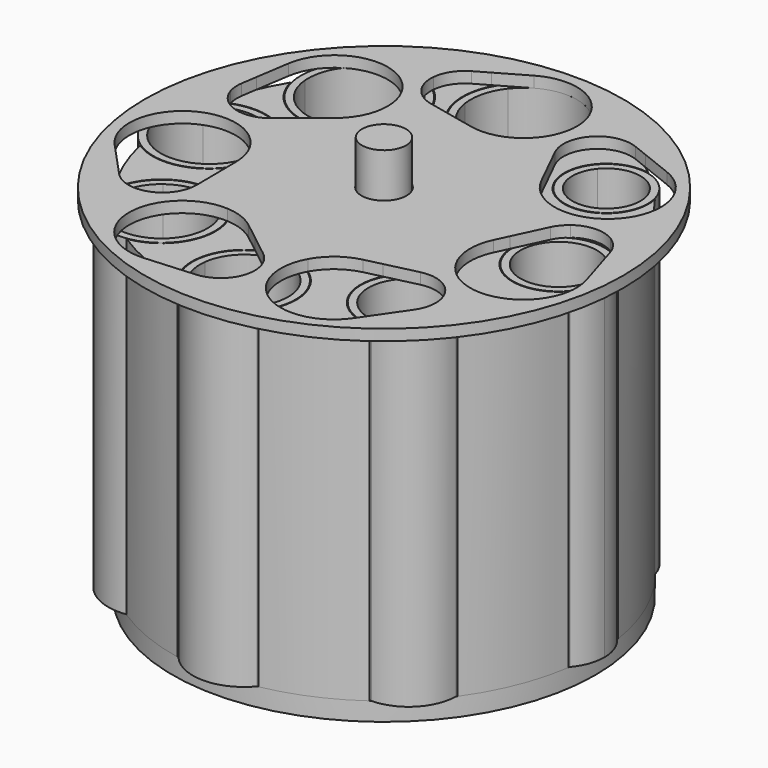
from build123d import *

# Parameters (mm, degrees)
F1_DEPTH = 90
F3_START = -90
F2_R     = 57.5
F2_R_2   = 6
F3_DEPTH = 5
F4_DEPTH = 90
F5_DEPTH = 88
F6_R     = 65
F6_R_2   = 6.125
F7_DEPTH = 3
F8_DEPTH = 15


with BuildPart() as f1:
    # F0 (on Top) → F1 (new body)
    with BuildSketch(Plane.XY):
        with BuildLine():
            ThreePointArc((45.8288421053, -12.4886841297), (34.9, 0), (45.8288421053, 12.4886841297))
            ThreePointArc((45.8288421053, 12.4886841297), (43.6591869219, 18.7116380181), (40.6490973012, 24.5743949793))
            ThreePointArc((40.6490973012, 24.5743949793), (25.4911994618, 25.4911994618), (24.5743949793, 40.6490973012))
            ThreePointArc((24.5743949793, 40.6490973012), (20.5775093162, 42.8114016396), (16.3922850173, 44.5818684211))
            ThreePointArc((16.3922850173, 44.5818684211), (0, 30.85), (-16.3922850173, 44.5818684211))
            ThreePointArc((-16.3922850173, 44.5818684211), (-18.4350753796, 43.7766832429), (-20.4384723604, 42.8779529312))
            ThreePointArc((-20.4384723604, 42.8779529312), (-22.2031529293, 22.2031529293), (-42.8779529312, 20.4384723604))
            ThreePointArc((-42.8779529312, 20.4384723604), (-44.0188706587, 17.8490623265), (-45.0035789474, 15.196311458))
            ThreePointArc((-45.0035789474, 15.196311458), (-32.1, 0), (-45.0035789474, -15.196311458))
            ThreePointArc((-45.0035789474, -15.196311458), (-43.7474044611, -18.5044481928), (-42.2484404987, -21.7098888857))
            ThreePointArc((-42.2484404987, -21.7098888857), (-23.1931024229, -23.1931024229), (-21.7098888857, -42.2484404987))
            ThreePointArc((-21.7098888857, -42.2484404987), (-17.9271288895, -43.9871350485), (-14.0066541239, -45.3879239474))
            ThreePointArc((-14.0066541239, -45.3879239474), (0, -33.335), (14.0066541239, -45.3879239474))
            ThreePointArc((14.0066541239, -45.3879239474), (18.6501874241, -43.6854725171), (23.0915279575, -41.5094126264))
            ThreePointArc((23.0915279575, -41.5094126264), (24.2891179338, -24.2891179338), (41.5094126264, -23.0915279575))
            ThreePointArc((41.5094126264, -23.0915279575), (43.9897460689, -17.9207209899), (45.8288421053, -12.4886841297))
        make_face()
        with BuildLine():
            ThreePointArc((-45.0035789474, 15.196311458), (-44.0188706587, 17.8490623265), (-42.8779529312, 20.4384723604))
            ThreePointArc((-42.8779529312, 20.4384723604), (-46.8858301809, 24.5119821981), (-49.2183268695, 29.728879901))
            ThreePointArc((-49.2183268695, 29.728879901), (-53.3131505624, 21.5396837746), (-56.0562105263, 12.804345412))
            ThreePointArc((-56.0562105263, 12.804345412), (-50.7573973518, 15.0515568129), (-45.0035789474, 15.196311458))
        make_face()
        with BuildLine():
            ThreePointArc((-20.4384723604, 42.8779529312), (-18.4350753796, 43.7766832429), (-16.3922850173, 44.5818684211))
            ThreePointArc((-16.3922850173, 44.5818684211), (-16.4179978261, 50.2698099905), (-14.5276429523, 55.6345))
            ThreePointArc((-14.5276429523, 55.6345), (-22.3596013645, 52.974505442), (-29.728879901, 49.2183268695))
            ThreePointArc((-29.728879901, 49.2183268695), (-24.5119821981, 46.8858301809), (-20.4384723604, 42.8779529312))
        make_face()
        with BuildLine():
            ThreePointArc((16.3922850173, 44.5818684211), (20.5775093162, 42.8114016396), (24.5743949793, 40.6490973012))
            ThreePointArc((24.5743949793, 40.6490973012), (29.7395661179, 44.3716042796), (36.0945159972, 44.7597577622))
            ThreePointArc((36.0945159972, 44.7597577622), (25.8885254285, 51.3423241696), (14.5276429523, 55.6345))
            ThreePointArc((14.5276429523, 55.6345), (16.4179978261, 50.2698099905), (16.3922850173, 44.5818684211))
        make_face()
        with BuildLine():
            ThreePointArc((40.6490973012, 24.5743949793), (43.6591869219, 18.7116380181), (45.8288421053, 12.4886841297))
            ThreePointArc((45.8288421053, 12.4886841297), (51.861049423, 11.8212202386), (56.8814736842, 8.4111801498))
            ThreePointArc((56.8814736842, 8.4111801498), (52.6718782026, 23.0634612885), (44.7597577622, 36.0945159972))
            ThreePointArc((44.7597577622, 36.0945159972), (44.3716042796, 29.7395661179), (40.6490973012, 24.5743949793))
        make_face()
        with BuildLine():
            ThreePointArc((56.8814736842, -8.4111801498), (51.861049423, -11.8212202386), (45.8288421053, -12.4886841297))
            ThreePointArc((45.8288421053, -12.4886841297), (43.9897460689, -17.9207209899), (41.5094126264, -23.0915279575))
            ThreePointArc((41.5094126264, -23.0915279575), (45.3373590848, -27.6829124242), (46.7372425875, -33.4944794753))
            ThreePointArc((46.7372425875, -33.4944794753), (53.3057460947, -21.558001607), (56.8814736842, -8.4111801498))
        make_face()
        with BuildLine():
            ThreePointArc((33.4944794753, -46.7372425875), (27.6829124242, -45.3373590848), (23.0915279575, -41.5094126264))
            ThreePointArc((23.0915279575, -41.5094126264), (18.6501874241, -43.6854725171), (14.0066541239, -45.3879239474))
            ThreePointArc((14.0066541239, -45.3879239474), (13.6642080444, -51.2331814208), (10.9869782871, -56.4405555263))
            ThreePointArc((10.9869782871, -56.4405555263), (22.7637560974, -52.8020966282), (33.4944794753, -46.7372425875))
        make_face()
        with BuildLine():
            ThreePointArc((-10.9869782871, -56.4405555263), (-13.6642080444, -51.2331814208), (-14.0066541239, -45.3879239474))
            ThreePointArc((-14.0066541239, -45.3879239474), (-17.9271288895, -43.9871350485), (-21.7098888857, -42.2484404987))
            ThreePointArc((-21.7098888857, -42.2484404987), (-25.9905791148, -46.1723127666), (-31.4567884644, -48.1323223989))
            ThreePointArc((-31.4567884644, -48.1323223989), (-21.6246391516, -53.2787479354), (-10.9869782871, -56.4405555263))
        make_face()
        with BuildLine():
            ThreePointArc((-48.1323223989, -31.4567884644), (-46.1723127666, -25.9905791148), (-42.2484404987, -21.7098888857))
            ThreePointArc((-42.2484404987, -21.7098888857), (-43.7474044611, -18.5044481928), (-45.0035789474, -15.196311458))
            ThreePointArc((-45.0035789474, -15.196311458), (-50.7573973518, -15.0515568129), (-56.0562105263, -12.804345412))
            ThreePointArc((-56.0562105263, -12.804345412), (-52.9224999998, -22.4824152121), (-48.1323223989, -31.4567884644))
        make_face()
    extrude(amount=-F1_DEPTH)

    # F2 (on face) → F3 (join)
    with BuildSketch(Plane.XY.offset(F3_START)):
        Circle(F2_R)
        Circle(F2_R_2, mode=Mode.SUBTRACT)
    extrude(amount=-F3_DEPTH)

    # F2 (on face) → F8 (join)
    with BuildSketch(Plane.XY):
        Circle(F2_R_2)
    extrude(amount=F8_DEPTH)


with BuildPart() as f4:
    # F0 (on Top) → F4 (new body)
    with BuildSketch(Plane.XY):
        with BuildLine():
            ThreePointArc((46.3614736842, -10.3374928212), (47.2145104814, -5.2), (47.5, 0))
            ThreePointArc((47.5, 0), (47.2145104814, 5.2), (46.3614736842, 10.3374928212))
            ThreePointArc((46.3614736842, 10.3374928212), (37.1, 0), (46.3614736842, -10.3374928212))
        make_face()
        with BuildLine():
            ThreePointArc((46.3614736842, 10.3374928212), (47.2145104814, 5.2), (47.5, 0))
            ThreePointArc((47.5, 0), (47.2145104814, -5.2), (46.3614736842, -10.3374928212))
            ThreePointArc((46.3614736842, -10.3374928212), (53.1742769409, -8.7156515074), (57.4141052632, -3.141737868))
            ThreePointArc((57.4141052632, -3.141737868), (57.4785223046, -1.5714559123), (57.5, 0))
            ThreePointArc((57.5, 0), (57.4785223046, 1.5714559123), (57.4141052632, 3.141737868))
            ThreePointArc((57.4141052632, 3.141737868), (53.1742769409, 8.7156515074), (46.3614736842, 10.3374928212))
        make_face()
        with BuildLine():
            ThreePointArc((46.3614736842, -10.3374928212), (37.1, 0), (46.3614736842, 10.3374928212))
            ThreePointArc((46.3614736842, 10.3374928212), (46.1318461889, 11.3182492995), (45.8814736842, 12.2939160793))
            ThreePointArc((45.8814736842, 12.2939160793), (35.1, 0), (45.8814736842, -12.2939160793))
            ThreePointArc((45.8814736842, -12.2939160793), (46.1318461889, -11.3182492995), (46.3614736842, -10.3374928212))
        make_face()
        with BuildLine():
            ThreePointArc((45.8814736842, 12.2939160793), (46.1318461889, 11.3182492995), (46.3614736842, 10.3374928212))
            ThreePointArc((46.3614736842, 10.3374928212), (53.1742769409, 8.7156515074), (57.4141052632, 3.141737868))
            ThreePointArc((57.4141052632, 3.141737868), (57.2266916516, 5.5996216495), (56.9341052632, 8.0472142934))
            ThreePointArc((56.9341052632, 8.0472142934), (51.9474079625, 11.5749972965), (45.8814736842, 12.2939160793))
        make_face()
        with BuildLine():
            ThreePointArc((57.4141052632, -3.141737868), (53.1742769409, -8.7156515074), (46.3614736842, -10.3374928212))
            ThreePointArc((46.3614736842, -10.3374928212), (46.1318461889, -11.3182492995), (45.8814736842, -12.2939160793))
            ThreePointArc((45.8814736842, -12.2939160793), (51.9474079625, -11.5749972965), (56.9341052632, -8.0472142934))
            ThreePointArc((56.9341052632, -8.0472142934), (57.2266916516, -5.5996216495), (57.4141052632, -3.141737868))
        make_face()
        with BuildLine():
            ThreePointArc((56.9341052632, 8.0472142934), (57.2266916516, 5.5996216495), (57.4141052632, 3.141737868))
            ThreePointArc((57.4141052632, 3.141737868), (57.7778084905, 1.5895447875), (57.9, 0))
            ThreePointArc((57.9, 0), (57.7778084905, -1.5895447875), (57.4141052632, -3.141737868))
            ThreePointArc((57.4141052632, -3.141737868), (57.2266916516, -5.5996216495), (56.9341052632, -8.0472142934))
            ThreePointArc((56.9341052632, -8.0472142934), (59.1349238344, -4.2881869559), (59.9, 0))
            ThreePointArc((59.9, 0), (59.1349238344, 4.2881869559), (56.9341052632, 8.0472142934))
        make_face()
        with BuildLine():
            ThreePointArc((57.9, 0), (57.7778084905, 1.5895447875), (57.4141052632, 3.141737868))
            ThreePointArc((57.4141052632, 3.141737868), (57.4785223046, 1.5714559123), (57.5, 0))
            ThreePointArc((57.5, 0), (57.4785223046, -1.5714559123), (57.4141052632, -3.141737868))
            ThreePointArc((57.4141052632, -3.141737868), (57.7778084905, -1.5895447875), (57.9, 0))
        make_face()
    extrude(amount=-F4_DEPTH)


with BuildPart() as f4b:
    # F0 (on Top) → F4, piece 2 (new body)
    with BuildSketch(Plane.XY):
        with BuildLine():
            ThreePointArc((24.74656236, 40.5445144423), (25.632620818, 25.632620818), (40.5445144423, 24.74656236))
            ThreePointArc((40.5445144423, 24.74656236), (40.0114132649, 25.5995470378), (39.4603696004, 26.4410520025))
            ThreePointArc((39.4603696004, 26.4410520025), (27.0468343804, 27.0468343804), (26.4410520025, 39.4603696004))
            ThreePointArc((26.4410520025, 39.4603696004), (25.5995470378, 40.0114132649), (24.74656236, 40.5445144423))
        make_face()
        with BuildLine():
            ThreePointArc((39.4603696004, 26.4410520025), (40.0114132649, 25.5995470378), (40.5445144423, 24.74656236))
            ThreePointArc((40.5445144423, 24.74656236), (43.7075548455, 28.673464928), (44.8375721064, 33.5875721064))
            ThreePointArc((44.8375721064, 33.5875721064), (44.7442174743, 35.0338653457), (44.465702927, 36.4561553542))
            ThreePointArc((44.465702927, 36.4561553542), (40.6586399182, 40.6586399182), (36.4561553542, 44.465702927))
            ThreePointArc((36.4561553542, 44.465702927), (30.01526202, 44.2553319765), (24.74656236, 40.5445144423))
            ThreePointArc((24.74656236, 40.5445144423), (25.5995470378, 40.0114132649), (26.4410520025, 39.4603696004))
            ThreePointArc((26.4410520025, 39.4603696004), (36.7066416022, 42.295838609), (42.8375721064, 33.5875721064))
            ThreePointArc((42.8375721064, 33.5875721064), (41.9507615942, 29.6354130015), (39.4603696004, 26.4410520025))
        make_face()
        with BuildLine():
            ThreePointArc((26.4410520025, 39.4603696004), (27.0468343804, 27.0468343804), (39.4603696004, 26.4410520025))
            ThreePointArc((39.4603696004, 26.4410520025), (33.5875721064, 33.5875721064), (26.4410520025, 39.4603696004))
        make_face()
        with BuildLine():
            ThreePointArc((26.4410520025, 39.4603696004), (33.5875721064, 33.5875721064), (39.4603696004, 26.4410520025))
            ThreePointArc((39.4603696004, 26.4410520025), (41.9507615942, 29.6354130015), (42.8375721064, 33.5875721064))
            ThreePointArc((42.8375721064, 33.5875721064), (36.7066416022, 42.295838609), (26.4410520025, 39.4603696004))
        make_face()
        with BuildLine():
            ThreePointArc((36.4561553542, 44.465702927), (40.6586399182, 40.6586399182), (44.465702927, 36.4561553542))
            ThreePointArc((44.465702927, 36.4561553542), (41.5425233947, 41.5425233947), (36.4561553542, 44.465702927))
        make_face()
    extrude(amount=-F4_DEPTH)


with BuildPart() as f4c:
    # F0 (on Top) → F4, piece 3 (new body)
    with BuildSketch(Plane.XY):
        with BuildLine():
            ThreePointArc((46.5375721064, -33.5875721064), (45.1852946269, -27.8260330467), (41.4108798537, -23.2677680438))
            ThreePointArc((41.4108798537, -23.2677680438), (40.9078129367, -24.1412684161), (40.3863236025, -25.0038970138))
            ThreePointArc((40.3863236025, -25.0038970138), (43.4452804831, -28.8201739104), (44.5375721064, -33.5875721064))
            ThreePointArc((44.5375721064, -33.5875721064), (44.3968014713, -35.3377322523), (43.9781089947, -37.0428931004))
            ThreePointArc((43.9781089947, -37.0428931004), (45.2866941674, -35.4311350564), (46.5362418024, -33.7731875739))
            ThreePointArc((46.5362418024, -33.7731875739), (46.5372395261, -33.6803822237), (46.5375721064, -33.5875721064))
        make_face()
        with BuildLine():
            ThreePointArc((40.3863236025, -25.0038970138), (40.9078129367, -24.1412684161), (41.4108798537, -23.2677680438))
            ThreePointArc((41.4108798537, -23.2677680438), (24.43053929, -24.43053929), (23.2677680438, -41.4108798537))
            ThreePointArc((23.2677680438, -41.4108798537), (24.1412684161, -40.9078129367), (25.0038970138, -40.3863236025))
            ThreePointArc((25.0038970138, -40.3863236025), (25.8447528524, -25.8447528524), (40.3863236025, -25.0038970138))
        make_face()
        with BuildLine():
            ThreePointArc((44.5375721064, -33.5875721064), (43.4452804831, -28.8201739104), (40.3863236025, -25.0038970138))
            ThreePointArc((40.3863236025, -25.0038970138), (33.5875721064, -33.5875721064), (25.0038970138, -40.3863236025))
            ThreePointArc((25.0038970138, -40.3863236025), (30.4570394814, -44.0805347711), (37.0428931004, -43.9781089947))
            ThreePointArc((37.0428931004, -43.9781089947), (40.6586399182, -40.6586399182), (43.9781089947, -37.0428931004))
            ThreePointArc((43.9781089947, -37.0428931004), (44.3968014713, -35.3377322523), (44.5375721064, -33.5875721064))
        make_face()
        with BuildLine():
            ThreePointArc((25.0038970138, -40.3863236025), (33.5875721064, -33.5875721064), (40.3863236025, -25.0038970138))
            ThreePointArc((40.3863236025, -25.0038970138), (25.8447528524, -25.8447528524), (25.0038970138, -40.3863236025))
        make_face()
        with BuildLine():
            ThreePointArc((25.0038970138, -40.3863236025), (24.1412684161, -40.9078129367), (23.2677680438, -41.4108798537))
            ThreePointArc((23.2677680438, -41.4108798537), (27.9092996229, -45.2262885993), (33.7731875739, -46.5362418024))
            ThreePointArc((33.7731875739, -46.5362418024), (35.4311350564, -45.2866941674), (37.0428931004, -43.9781089947))
            ThreePointArc((37.0428931004, -43.9781089947), (30.4570394814, -44.0805347711), (25.0038970138, -40.3863236025))
        make_face()
        with BuildLine():
            ThreePointArc((33.7731875739, -46.5362418024), (42.7446049227, -42.7446049227), (46.5362418024, -33.7731875739))
            ThreePointArc((46.5362418024, -33.7731875739), (45.2866941674, -35.4311350564), (43.9781089947, -37.0428931004))
            ThreePointArc((43.9781089947, -37.0428931004), (41.3303913604, -41.3303913604), (37.0428931004, -43.9781089947))
            ThreePointArc((37.0428931004, -43.9781089947), (35.4311350564, -45.2866941674), (33.7731875739, -46.5362418024))
        make_face()
        with BuildLine():
            ThreePointArc((37.0428931004, -43.9781089947), (41.3303913604, -41.3303913604), (43.9781089947, -37.0428931004))
            ThreePointArc((43.9781089947, -37.0428931004), (40.6586399182, -40.6586399182), (37.0428931004, -43.9781089947))
        make_face()
    extrude(amount=-F4_DEPTH)


with BuildPart() as f4d:
    # F0 (on Top) → F4, piece 4 (new body)
    with BuildSketch(Plane.XY):
        with BuildLine():
            ThreePointArc((-16.2015075715, 44.6515526316), (0, 31.05), (16.2015075715, 44.6515526316))
            ThreePointArc((16.2015075715, 44.6515526316), (15.2451560735, 44.9870560972), (14.2818641307, 45.3020789474))
            ThreePointArc((14.2818641307, 45.3020789474), (0, 33.05), (-14.2818641307, 45.3020789474))
            ThreePointArc((-14.2818641307, 45.3020789474), (-15.2451560735, 44.9870560972), (-16.2015075715, 44.6515526316))
        make_face()
        with BuildLine():
            ThreePointArc((14.2818641307, 45.3020789474), (15.2451560735, 44.9870560972), (16.2015075715, 44.6515526316))
            ThreePointArc((16.2015075715, 44.6515526316), (16.3877591444, 46.0703671015), (16.45, 47.5))
            ThreePointArc((16.45, 47.5), (15.8925847832, 51.7459685477), (14.2581156343, 55.7041842105))
            ThreePointArc((14.2581156343, 55.7041842105), (12.8427439505, 56.047425702), (11.4191331324, 56.3547105263))
            ThreePointArc((11.4191331324, 56.3547105263), (13.6713015796, 52.1795312926), (14.45, 47.5))
            ThreePointArc((14.45, 47.5), (14.4079047173, 46.397828663), (14.2818641307, 45.3020789474))
        make_face()
        with BuildLine():
            ThreePointArc((-14.2818641307, 45.3020789474), (0, 33.05), (14.2818641307, 45.3020789474))
            ThreePointArc((14.2818641307, 45.3020789474), (0, 47.5), (-14.2818641307, 45.3020789474))
        make_face()
        with BuildLine():
            ThreePointArc((-14.2818641307, 45.3020789474), (0, 47.5), (14.2818641307, 45.3020789474))
            ThreePointArc((14.2818641307, 45.3020789474), (14.4079047173, 46.397828663), (14.45, 47.5))
            ThreePointArc((14.45, 47.5), (13.6713015796, 52.1795312926), (11.4191331324, 56.3547105263))
            ThreePointArc((11.4191331324, 56.3547105263), (0, 57.5), (-11.4191331324, 56.3547105263))
            ThreePointArc((-11.4191331324, 56.3547105263), (-13.9884052445, 51.1231227852), (-14.2818641307, 45.3020789474))
        make_face()
        with BuildLine():
            ThreePointArc((-14.2581156343, 55.7041842105), (-16.2014606645, 50.3487141548), (-16.2015075715, 44.6515526316))
            ThreePointArc((-16.2015075715, 44.6515526316), (-15.2451560735, 44.9870560972), (-14.2818641307, 45.3020789474))
            ThreePointArc((-14.2818641307, 45.3020789474), (-13.9884052445, 51.1231227852), (-11.4191331324, 56.3547105263))
            ThreePointArc((-11.4191331324, 56.3547105263), (-12.8427439505, 56.047425702), (-14.2581156343, 55.7041842105))
        make_face()
        with BuildLine():
            ThreePointArc((11.4191331324, 56.3547105263), (12.8427439505, 56.047425702), (14.2581156343, 55.7041842105))
            ThreePointArc((14.2581156343, 55.7041842105), (0, 63.95), (-14.2581156343, 55.7041842105))
            ThreePointArc((-14.2581156343, 55.7041842105), (-12.8427439505, 56.047425702), (-11.4191331324, 56.3547105263))
            ThreePointArc((-11.4191331324, 56.3547105263), (0, 61.95), (11.4191331324, 56.3547105263))
        make_face()
        with BuildLine():
            ThreePointArc((-11.4191331324, 56.3547105263), (0, 57.5), (11.4191331324, 56.3547105263))
            ThreePointArc((11.4191331324, 56.3547105263), (0, 61.95), (-11.4191331324, 56.3547105263))
        make_face()
    extrude(amount=-F4_DEPTH)


with BuildPart() as f4e:
    # F0 (on Top) → F4, piece 5 (new body)
    with BuildSketch(Plane.XY):
        with BuildLine():
            ThreePointArc((13.965, -47.5), (13.9270211349, -46.4707734412), (13.8132911121, -45.447145))
            ThreePointArc((13.8132911122, -45.447145), (12.8444068922, -45.7304188871), (11.8697218066, -45.9930397368))
            ThreePointArc((11.8697218066, -45.9930397368), (11.9411566947, -46.7450153695), (11.965, -47.5))
            ThreePointArc((11.965, -47.5), (10.7115916987, -52.8313251898), (7.2139714534, -57.0456713158))
            ThreePointArc((7.2139714534, -57.0456713158), (8.950278823, -56.799141798), (10.6782604636, -56.4997765789))
            ThreePointArc((10.6782604636, -56.4997765789), (13.1176052002, -52.2905802167), (13.965, -47.5))
        make_face()
        with BuildLine():
            ThreePointArc((11.8697218066, -45.9930397368), (12.8444068922, -45.7304188871), (13.8132911122, -45.447145))
            ThreePointArc((13.8132911121, -45.447145), (0, -33.535), (-13.8132911121, -45.447145))
            ThreePointArc((-13.8132911122, -45.447145), (-12.8444068922, -45.7304188871), (-11.8697218066, -45.9930397368))
            ThreePointArc((-11.8697218066, -45.9930397368), (0, -35.535), (11.8697218066, -45.9930397368))
        make_face()
        with BuildLine():
            ThreePointArc((11.965, -47.5), (11.9411566947, -46.7450153695), (11.8697218066, -45.9930397368))
            ThreePointArc((11.8697218066, -45.9930397368), (0, -47.5), (-11.8697218066, -45.9930397368))
            ThreePointArc((-11.8697218066, -45.9930397368), (-11.0266496868, -52.1448058823), (-7.2139714534, -57.0456713158))
            ThreePointArc((-7.2139714534, -57.0456713158), (0, -57.5), (7.2139714534, -57.0456713158))
            ThreePointArc((7.2139714534, -57.0456713158), (10.7115916987, -52.8313251898), (11.965, -47.5))
        make_face()
        with BuildLine():
            ThreePointArc((-11.8697218066, -45.9930397368), (0, -47.5), (11.8697218066, -45.9930397368))
            ThreePointArc((11.8697218066, -45.9930397368), (0, -35.535), (-11.8697218066, -45.9930397368))
        make_face()
        with BuildLine():
            ThreePointArc((-11.8697218066, -45.9930397368), (-12.8444068922, -45.7304188871), (-13.8132911122, -45.447145))
            ThreePointArc((-13.8132911121, -45.447145), (-13.4349987291, -51.31077868), (-10.6782604636, -56.4997765789))
            ThreePointArc((-10.6782604636, -56.4997765789), (-8.950278823, -56.799141798), (-7.2139714534, -57.0456713158))
            ThreePointArc((-7.2139714534, -57.0456713158), (-11.0266496868, -52.1448058823), (-11.8697218066, -45.9930397368))
        make_face()
        with BuildLine():
            ThreePointArc((-10.6782604636, -56.4997765789), (0, -61.465), (10.6782604636, -56.4997765789))
            ThreePointArc((10.6782604636, -56.4997765789), (8.950278823, -56.799141798), (7.2139714534, -57.0456713158))
            ThreePointArc((7.2139714534, -57.0456713158), (0, -59.465), (-7.2139714534, -57.0456713158))
            ThreePointArc((-7.2139714534, -57.0456713158), (-8.950278823, -56.799141798), (-10.6782604636, -56.4997765789))
        make_face()
        with BuildLine():
            ThreePointArc((-7.2139714534, -57.0456713158), (0, -59.465), (7.2139714534, -57.0456713158))
            ThreePointArc((7.2139714534, -57.0456713158), (0, -57.5), (-7.2139714534, -57.0456713158))
        make_face()
    extrude(amount=-F4_DEPTH)


with BuildPart() as f4f:
    # F0 (on Top) → F4, piece 6 (new body)
    with BuildSketch(Plane.XY):
        with BuildLine():
            ThreePointArc((-17.6875721064, 33.5875721064), (-18.4387851423, 38.41709108), (-20.6214404733, 42.7902581531))
            ThreePointArc((-20.6214404733, 42.7902581531), (-21.5288412802, 42.3409847917), (-22.426459546, 41.8724720101))
            ThreePointArc((-22.426459546, 41.8724720101), (-20.3900445995, 37.9505146576), (-19.6875721064, 33.5875721064))
            ThreePointArc((-19.6875721064, 33.5875721064), (-27.3405771753, 21.1704446475), (-41.8724720101, 22.426459546))
            ThreePointArc((-41.8724720101, 22.426459546), (-42.3409847917, 21.5288412802), (-42.7902581531, 20.6214404733))
            ThreePointArc((-42.7902581531, 20.6214404733), (-26.2907477335, 19.4607765012), (-17.6875721064, 33.5875721064))
        make_face()
        with BuildLine():
            ThreePointArc((-22.426459546, 41.8724720101), (-21.5288412802, 42.3409847917), (-20.6214404733, 42.7902581531))
            ThreePointArc((-20.6214404733, 42.7902581531), (-24.7217011138, 46.7862967244), (-29.971549759, 49.0709303462))
            ThreePointArc((-29.971549759, 49.0709303462), (-31.2393048097, 48.2737592798), (-32.4858697184, 47.4438433165))
            ThreePointArc((-32.4858697184, 47.4438433165), (-26.8530192502, 45.7471690498), (-22.426459546, 41.8724720101))
        make_face()
        with BuildLine():
            ThreePointArc((-19.6875721064, 33.5875721064), (-20.3900445995, 37.9505146576), (-22.426459546, 41.8724720101))
            ThreePointArc((-22.426459546, 41.8724720101), (-33.5875721064, 33.5875721064), (-41.8724720101, 22.426459546))
            ThreePointArc((-41.8724720101, 22.426459546), (-27.3405771753, 21.1704446475), (-19.6875721064, 33.5875721064))
        make_face()
        with BuildLine():
            ThreePointArc((-41.8724720101, 22.426459546), (-33.5875721064, 33.5875721064), (-22.426459546, 41.8724720101))
            ThreePointArc((-22.426459546, 41.8724720101), (-26.8530192502, 45.7471690498), (-32.4858697184, 47.4438433165))
            ThreePointArc((-32.4858697184, 47.4438433165), (-40.6586399182, 40.6586399182), (-47.4438433165, 32.4858697184))
            ThreePointArc((-47.4438433165, 32.4858697184), (-45.7471690498, 26.8530192502), (-41.8724720101, 22.426459546))
        make_face()
        with BuildLine():
            ThreePointArc((-32.4858697184, 47.4438433165), (-31.2393048097, 48.2737592798), (-29.971549759, 49.0709303462))
            ThreePointArc((-29.971549759, 49.0709303462), (-44.8305699272, 44.8305699272), (-49.0709303462, 29.971549759))
            ThreePointArc((-49.0709303462, 29.971549759), (-48.2737592798, 31.2393048097), (-47.4438433165, 32.4858697184))
            ThreePointArc((-47.4438433165, 32.4858697184), (-43.4163563649, 43.4163563649), (-32.4858697184, 47.4438433165))
        make_face()
        with BuildLine():
            ThreePointArc((-49.0709303462, 29.971549759), (-46.7862967244, 24.7217011138), (-42.7902581531, 20.6214404733))
            ThreePointArc((-42.7902581531, 20.6214404733), (-42.3409847917, 21.5288412802), (-41.8724720101, 22.426459546))
            ThreePointArc((-41.8724720101, 22.426459546), (-45.7471690498, 26.8530192502), (-47.4438433165, 32.4858697184))
            ThreePointArc((-47.4438433165, 32.4858697184), (-48.2737592798, 31.2393048097), (-49.0709303462, 29.971549759))
        make_face()
        with BuildLine():
            ThreePointArc((-47.4438433165, 32.4858697184), (-40.6586399182, 40.6586399182), (-32.4858697184, 47.4438433165))
            ThreePointArc((-32.4858697184, 47.4438433165), (-43.4163563649, 43.4163563649), (-47.4438433165, 32.4858697184))
        make_face()
    extrude(amount=-F4_DEPTH)


with BuildPart() as f4g:
    # F0 (on Top) → F4, piece 7 (new body)
    with BuildSketch(Plane.XY):
        with BuildLine():
            ThreePointArc((-31.7104872101, -47.9655605711), (-26.2045644386, -46.0672034221), (-21.8897181675, -42.1555481348))
            ThreePointArc((-21.8897181675, -42.1555481348), (-22.7813017805, -41.6804785143), (-23.662580294, -41.1865547701))
            ThreePointArc((-23.662580294, -41.1865547701), (-28.4295298508, -44.9737303737), (-34.4200993118, -46.0598172311))
            ThreePointArc((-34.4200993118, -46.0598172311), (-33.0790202825, -47.0322061693), (-31.7104872101, -47.9655605711))
        make_face()
        with BuildLine():
            ThreePointArc((-23.662580294, -41.1865547701), (-22.7813017805, -41.6804785143), (-21.8897181675, -42.1555481348))
            ThreePointArc((-21.8897181675, -42.1555481348), (-19.8059016323, -38.0948505472), (-19.0875721064, -33.5875721064))
            ThreePointArc((-19.0875721064, -33.5875721064), (-27.0295866082, -20.6553323078), (-42.1555481348, -21.8897181675))
            ThreePointArc((-42.1555481348, -21.8897181675), (-41.6804785143, -22.7813017805), (-41.1865547701, -23.662580294))
            ThreePointArc((-41.1865547701, -23.662580294), (-28.0530117488, -22.3795998701), (-21.0875721064, -33.5875721064))
            ThreePointArc((-21.0875721064, -33.5875721064), (-21.748813775, -37.5992801182), (-23.662580294, -41.1865547701))
        make_face()
        with BuildLine():
            ThreePointArc((-34.4200993118, -46.0598172311), (-28.4295298508, -44.9737303737), (-23.662580294, -41.1865547701))
            ThreePointArc((-23.662580294, -41.1865547701), (-33.5875721064, -33.5875721064), (-41.1865547701, -23.662580294))
            ThreePointArc((-41.1865547701, -23.662580294), (-44.9737303737, -28.4295298508), (-46.0598172311, -34.4200993118))
            ThreePointArc((-46.0598172311, -34.4200993118), (-40.6586399182, -40.6586399182), (-34.4200993118, -46.0598172311))
        make_face()
        with BuildLine():
            ThreePointArc((-41.1865547701, -23.662580294), (-33.5875721064, -33.5875721064), (-23.662580294, -41.1865547701))
            ThreePointArc((-23.662580294, -41.1865547701), (-21.748813775, -37.5992801182), (-21.0875721064, -33.5875721064))
            ThreePointArc((-21.0875721064, -33.5875721064), (-28.0530117488, -22.3795998701), (-41.1865547701, -23.662580294))
        make_face()
        with BuildLine():
            ThreePointArc((-47.9655605711, -31.7104872101), (-43.8406204336, -43.8406204336), (-31.7104872101, -47.9655605711))
            ThreePointArc((-31.7104872101, -47.9655605711), (-33.0790202825, -47.0322061693), (-34.4200993118, -46.0598172311))
            ThreePointArc((-34.4200993118, -46.0598172311), (-42.4264068712, -42.4264068712), (-46.0598172311, -34.4200993118))
            ThreePointArc((-46.0598172311, -34.4200993118), (-47.0322061693, -33.0790202825), (-47.9655605711, -31.7104872101))
        make_face()
        with BuildLine():
            ThreePointArc((-41.1865547701, -23.662580294), (-41.6804785143, -22.7813017805), (-42.1555481348, -21.8897181675))
            ThreePointArc((-42.1555481348, -21.8897181675), (-46.0672034221, -26.2045644386), (-47.9655605711, -31.7104872101))
            ThreePointArc((-47.9655605711, -31.7104872101), (-47.0322061693, -33.0790202825), (-46.0598172311, -34.4200993118))
            ThreePointArc((-46.0598172311, -34.4200993118), (-44.9737303737, -28.4295298508), (-41.1865547701, -23.662580294))
        make_face()
        with BuildLine():
            ThreePointArc((-46.0598172311, -34.4200993118), (-42.4264068712, -42.4264068712), (-34.4200993118, -46.0598172311))
            ThreePointArc((-34.4200993118, -46.0598172311), (-40.6586399182, -40.6586399182), (-46.0598172311, -34.4200993118))
        make_face()
    extrude(amount=-F4_DEPTH)


with BuildPart() as f4h:
    # F0 (on Top) → F4, piece 8 (new body)
    with BuildSketch(Plane.XY):
        with BuildLine():
            ThreePointArc((-32.3, 0), (-35.9240248791, 9.8507258616), (-45.068, 15.004178618))
            ThreePointArc((-45.068, 15.004178618), (-45.3772330987, 14.041250525), (-45.6658947368, 13.0719569263))
            ThreePointArc((-45.6658947368, 13.0719569263), (-37.5388206152, 8.6611145509), (-34.3, 0))
            ThreePointArc((-34.3, 0), (-37.5388206152, -8.6611145509), (-45.6658947368, -13.0719569263))
            ThreePointArc((-45.6658947368, -13.0719569263), (-45.3772330987, -14.041250525), (-45.068, -15.004178618))
            ThreePointArc((-45.068, -15.004178618), (-35.9240248791, -9.8507258616), (-32.3, 0))
        make_face()
        with BuildLine():
            ThreePointArc((-45.6658947368, 13.0719569263), (-45.3772330987, 14.041250525), (-45.068, 15.004178618))
            ThreePointArc((-45.068, 15.004178618), (-50.8344940614, 14.8297386813), (-56.1206315789, 12.5189740466))
            ThreePointArc((-56.1206315789, 12.5189740466), (-56.4404738731, 10.9873977348), (-56.7185263158, 9.4476860958))
            ThreePointArc((-56.7185263158, 9.4476860958), (-51.6129373122, 12.5428763315), (-45.6658947368, 13.0719569263))
        make_face()
        with BuildLine():
            ThreePointArc((-56.1206315789, -12.5189740466), (-50.8344940614, -14.8297386813), (-45.068, -15.004178618))
            ThreePointArc((-45.068, -15.004178618), (-45.3772330987, -14.041250525), (-45.6658947368, -13.0719569263))
            ThreePointArc((-45.6658947368, -13.0719569263), (-51.6129373122, -12.5428763315), (-56.7185263158, -9.4476860958))
            ThreePointArc((-56.7185263158, -9.4476860958), (-56.4404738731, -10.9873977348), (-56.1206315789, -12.5189740466))
        make_face()
        with BuildLine():
            ThreePointArc((-34.3, 0), (-37.5388206152, 8.6611145509), (-45.6658947368, 13.0719569263))
            ThreePointArc((-45.6658947368, 13.0719569263), (-47.5, 0), (-45.6658947368, -13.0719569263))
            ThreePointArc((-45.6658947368, -13.0719569263), (-37.5388206152, -8.6611145509), (-34.3, 0))
        make_face()
        with BuildLine():
            ThreePointArc((-45.6658947368, -13.0719569263), (-47.5, 0), (-45.6658947368, 13.0719569263))
            ThreePointArc((-45.6658947368, 13.0719569263), (-51.6129373122, 12.5428763315), (-56.7185263158, 9.4476860958))
            ThreePointArc((-56.7185263158, 9.4476860958), (-57.5, 0), (-56.7185263158, -9.4476860958))
            ThreePointArc((-56.7185263158, -9.4476860958), (-51.6129373122, -12.5428763315), (-45.6658947368, -13.0719569263))
        make_face()
        with BuildLine():
            ThreePointArc((-56.7185263158, 9.4476860958), (-56.4404738731, 10.9873977348), (-56.1206315789, 12.5189740466))
            ThreePointArc((-56.1206315789, 12.5189740466), (-62.7, 0), (-56.1206315789, -12.5189740466))
            ThreePointArc((-56.1206315789, -12.5189740466), (-56.4404738731, -10.9873977348), (-56.7185263158, -9.4476860958))
            ThreePointArc((-56.7185263158, -9.4476860958), (-60.7, 0), (-56.7185263158, 9.4476860958))
        make_face()
        with BuildLine():
            ThreePointArc((-56.7185263158, -9.4476860958), (-57.5, 0), (-56.7185263158, 9.4476860958))
            ThreePointArc((-56.7185263158, 9.4476860958), (-60.7, 0), (-56.7185263158, -9.4476860958))
        make_face()
    extrude(amount=-F4_DEPTH)


with BuildPart() as f5_tool:
    # F0 (on Top) → F5 (new body)
    with BuildSketch(Plane.XY):
        with BuildLine():
            ThreePointArc((37.0428931004, -43.9781089947), (41.3303913604, -41.3303913604), (43.9781089947, -37.0428931004))
            ThreePointArc((43.9781089947, -37.0428931004), (40.6586399182, -40.6586399182), (37.0428931004, -43.9781089947))
        make_face()
        with BuildLine():
            ThreePointArc((44.5375721064, -33.5875721064), (43.4452804831, -28.8201739104), (40.3863236025, -25.0038970138))
            ThreePointArc((40.3863236025, -25.0038970138), (33.5875721064, -33.5875721064), (25.0038970138, -40.3863236025))
            ThreePointArc((25.0038970138, -40.3863236025), (30.4570394814, -44.0805347711), (37.0428931004, -43.9781089947))
            ThreePointArc((37.0428931004, -43.9781089947), (40.6586399182, -40.6586399182), (43.9781089947, -37.0428931004))
            ThreePointArc((43.9781089947, -37.0428931004), (44.3968014713, -35.3377322523), (44.5375721064, -33.5875721064))
        make_face()
        with BuildLine():
            ThreePointArc((25.0038970138, -40.3863236025), (33.5875721064, -33.5875721064), (40.3863236025, -25.0038970138))
            ThreePointArc((40.3863236025, -25.0038970138), (25.8447528524, -25.8447528524), (25.0038970138, -40.3863236025))
        make_face()
        with BuildLine():
            ThreePointArc((-7.2139714534, -57.0456713158), (0, -59.465), (7.2139714534, -57.0456713158))
            ThreePointArc((7.2139714534, -57.0456713158), (0, -57.5), (-7.2139714534, -57.0456713158))
        make_face()
        with BuildLine():
            ThreePointArc((11.965, -47.5), (11.9411566947, -46.7450153695), (11.8697218066, -45.9930397368))
            ThreePointArc((11.8697218066, -45.9930397368), (0, -47.5), (-11.8697218066, -45.9930397368))
            ThreePointArc((-11.8697218066, -45.9930397368), (-11.0266496868, -52.1448058823), (-7.2139714534, -57.0456713158))
            ThreePointArc((-7.2139714534, -57.0456713158), (0, -57.5), (7.2139714534, -57.0456713158))
            ThreePointArc((7.2139714534, -57.0456713158), (10.7115916987, -52.8313251898), (11.965, -47.5))
        make_face()
        with BuildLine():
            ThreePointArc((-11.8697218066, -45.9930397368), (0, -47.5), (11.8697218066, -45.9930397368))
            ThreePointArc((11.8697218066, -45.9930397368), (0, -35.535), (-11.8697218066, -45.9930397368))
        make_face()
        with BuildLine():
            ThreePointArc((-46.0598172311, -34.4200993118), (-42.4264068712, -42.4264068712), (-34.4200993118, -46.0598172311))
            ThreePointArc((-34.4200993118, -46.0598172311), (-40.6586399182, -40.6586399182), (-46.0598172311, -34.4200993118))
        make_face()
        with BuildLine():
            ThreePointArc((-34.4200993118, -46.0598172311), (-28.4295298508, -44.9737303737), (-23.662580294, -41.1865547701))
            ThreePointArc((-23.662580294, -41.1865547701), (-33.5875721064, -33.5875721064), (-41.1865547701, -23.662580294))
            ThreePointArc((-41.1865547701, -23.662580294), (-44.9737303737, -28.4295298508), (-46.0598172311, -34.4200993118))
            ThreePointArc((-46.0598172311, -34.4200993118), (-40.6586399182, -40.6586399182), (-34.4200993118, -46.0598172311))
        make_face()
        with BuildLine():
            ThreePointArc((-41.1865547701, -23.662580294), (-33.5875721064, -33.5875721064), (-23.662580294, -41.1865547701))
            ThreePointArc((-23.662580294, -41.1865547701), (-21.748813775, -37.5992801182), (-21.0875721064, -33.5875721064))
            ThreePointArc((-21.0875721064, -33.5875721064), (-28.0530117488, -22.3795998701), (-41.1865547701, -23.662580294))
        make_face()
        with BuildLine():
            ThreePointArc((-56.7185263158, -9.4476860958), (-57.5, 0), (-56.7185263158, 9.4476860958))
            ThreePointArc((-56.7185263158, 9.4476860958), (-60.7, 0), (-56.7185263158, -9.4476860958))
        make_face()
        with BuildLine():
            ThreePointArc((-45.6658947368, -13.0719569263), (-47.5, 0), (-45.6658947368, 13.0719569263))
            ThreePointArc((-45.6658947368, 13.0719569263), (-51.6129373122, 12.5428763315), (-56.7185263158, 9.4476860958))
            ThreePointArc((-56.7185263158, 9.4476860958), (-57.5, 0), (-56.7185263158, -9.4476860958))
            ThreePointArc((-56.7185263158, -9.4476860958), (-51.6129373122, -12.5428763315), (-45.6658947368, -13.0719569263))
        make_face()
        with BuildLine():
            ThreePointArc((-34.3, 0), (-37.5388206152, 8.6611145509), (-45.6658947368, 13.0719569263))
            ThreePointArc((-45.6658947368, 13.0719569263), (-47.5, 0), (-45.6658947368, -13.0719569263))
            ThreePointArc((-45.6658947368, -13.0719569263), (-37.5388206152, -8.6611145509), (-34.3, 0))
        make_face()
        with BuildLine():
            ThreePointArc((-47.4438433165, 32.4858697184), (-40.6586399182, 40.6586399182), (-32.4858697184, 47.4438433165))
            ThreePointArc((-32.4858697184, 47.4438433165), (-43.4163563649, 43.4163563649), (-47.4438433165, 32.4858697184))
        make_face()
        with BuildLine():
            ThreePointArc((-41.8724720101, 22.426459546), (-33.5875721064, 33.5875721064), (-22.426459546, 41.8724720101))
            ThreePointArc((-22.426459546, 41.8724720101), (-26.8530192502, 45.7471690498), (-32.4858697184, 47.4438433165))
            ThreePointArc((-32.4858697184, 47.4438433165), (-40.6586399182, 40.6586399182), (-47.4438433165, 32.4858697184))
            ThreePointArc((-47.4438433165, 32.4858697184), (-45.7471690498, 26.8530192502), (-41.8724720101, 22.426459546))
        make_face()
        with BuildLine():
            ThreePointArc((-19.6875721064, 33.5875721064), (-20.3900445995, 37.9505146576), (-22.426459546, 41.8724720101))
            ThreePointArc((-22.426459546, 41.8724720101), (-33.5875721064, 33.5875721064), (-41.8724720101, 22.426459546))
            ThreePointArc((-41.8724720101, 22.426459546), (-27.3405771753, 21.1704446475), (-19.6875721064, 33.5875721064))
        make_face()
        with BuildLine():
            ThreePointArc((-11.4191331324, 56.3547105263), (0, 57.5), (11.4191331324, 56.3547105263))
            ThreePointArc((11.4191331324, 56.3547105263), (0, 61.95), (-11.4191331324, 56.3547105263))
        make_face()
        with BuildLine():
            ThreePointArc((-14.2818641307, 45.3020789474), (0, 47.5), (14.2818641307, 45.3020789474))
            ThreePointArc((14.2818641307, 45.3020789474), (14.4079047173, 46.397828663), (14.45, 47.5))
            ThreePointArc((14.45, 47.5), (13.6713015796, 52.1795312926), (11.4191331324, 56.3547105263))
            ThreePointArc((11.4191331324, 56.3547105263), (0, 57.5), (-11.4191331324, 56.3547105263))
            ThreePointArc((-11.4191331324, 56.3547105263), (-13.9884052445, 51.1231227852), (-14.2818641307, 45.3020789474))
        make_face()
        with BuildLine():
            ThreePointArc((-14.2818641307, 45.3020789474), (0, 33.05), (14.2818641307, 45.3020789474))
            ThreePointArc((14.2818641307, 45.3020789474), (0, 47.5), (-14.2818641307, 45.3020789474))
        make_face()
        with BuildLine():
            ThreePointArc((26.4410520025, 39.4603696004), (33.5875721064, 33.5875721064), (39.4603696004, 26.4410520025))
            ThreePointArc((39.4603696004, 26.4410520025), (41.9507615942, 29.6354130015), (42.8375721064, 33.5875721064))
            ThreePointArc((42.8375721064, 33.5875721064), (36.7066416022, 42.295838609), (26.4410520025, 39.4603696004))
        make_face()
        with BuildLine():
            ThreePointArc((26.4410520025, 39.4603696004), (27.0468343804, 27.0468343804), (39.4603696004, 26.4410520025))
            ThreePointArc((39.4603696004, 26.4410520025), (33.5875721064, 33.5875721064), (26.4410520025, 39.4603696004))
        make_face()
        with BuildLine():
            ThreePointArc((46.3614736842, -10.3374928212), (47.2145104814, -5.2), (47.5, 0))
            ThreePointArc((47.5, 0), (47.2145104814, 5.2), (46.3614736842, 10.3374928212))
            ThreePointArc((46.3614736842, 10.3374928212), (37.1, 0), (46.3614736842, -10.3374928212))
        make_face()
        with BuildLine():
            ThreePointArc((46.3614736842, 10.3374928212), (47.2145104814, 5.2), (47.5, 0))
            ThreePointArc((47.5, 0), (47.2145104814, -5.2), (46.3614736842, -10.3374928212))
            ThreePointArc((46.3614736842, -10.3374928212), (53.1742769409, -8.7156515074), (57.4141052632, -3.141737868))
            ThreePointArc((57.4141052632, -3.141737868), (57.4785223046, -1.5714559123), (57.5, 0))
            ThreePointArc((57.5, 0), (57.4785223046, 1.5714559123), (57.4141052632, 3.141737868))
            ThreePointArc((57.4141052632, 3.141737868), (53.1742769409, 8.7156515074), (46.3614736842, 10.3374928212))
        make_face()
        with BuildLine():
            ThreePointArc((57.9, 0), (57.7778084905, 1.5895447875), (57.4141052632, 3.141737868))
            ThreePointArc((57.4141052632, 3.141737868), (57.4785223046, 1.5714559123), (57.5, 0))
            ThreePointArc((57.5, 0), (57.4785223046, -1.5714559123), (57.4141052632, -3.141737868))
            ThreePointArc((57.4141052632, -3.141737868), (57.7778084905, -1.5895447875), (57.9, 0))
        make_face()
    extrude(amount=-F5_DEPTH)


with BuildPart() as f4_1:
    add(f4.part)

    # F5: cut by f5_tool
    add(f5_tool.part, mode=Mode.SUBTRACT)


with BuildPart() as f4b_1:
    add(f4b.part)

    # F5: cut by f5_tool
    add(f5_tool.part, mode=Mode.SUBTRACT)


with BuildPart() as f4c_1:
    add(f4c.part)

    # F5: cut by f5_tool
    add(f5_tool.part, mode=Mode.SUBTRACT)


with BuildPart() as f4d_1:
    add(f4d.part)

    # F5: cut by f5_tool
    add(f5_tool.part, mode=Mode.SUBTRACT)


with BuildPart() as f4e_1:
    add(f4e.part)

    # F5: cut by f5_tool
    add(f5_tool.part, mode=Mode.SUBTRACT)


with BuildPart() as f4f_1:
    add(f4f.part)

    # F5: cut by f5_tool
    add(f5_tool.part, mode=Mode.SUBTRACT)


with BuildPart() as f4g_1:
    add(f4g.part)

    # F5: cut by f5_tool
    add(f5_tool.part, mode=Mode.SUBTRACT)


with BuildPart() as f4h_1:
    add(f4h.part)

    # F5: cut by f5_tool
    add(f5_tool.part, mode=Mode.SUBTRACT)


with BuildPart() as f7:
    # F6 (on face) → F7 (new body)
    with BuildSketch(Plane.XY):
        Circle(F6_R)
        with BuildLine():
            ThreePointArc((-7.190167227, 60.0341132613), (14.2818641307, 49.6979210526), (-3.0888214898, 33.3839920018))
            Line((-3.0888214898, 33.3839920018), (-11.1692721652, 35.1521313864))
            ThreePointArc((-11.1692721652, 35.1521313864), (10.3779342642, 34.4799777109), (14.5276429523, 55.6345))
            ThreePointArc((14.5276429523, 55.6345), (24.6581746689, 51.9444359099), (33.9217510983, 46.4280605068))
            Line((33.9217510983, 46.4280605068), (42.45356383, 43.0521564844))
            ThreePointArc((42.45356383, 43.0521564844), (49.9674078685, 36.2627962284), (51.179599929, 26.2087495145))
            ThreePointArc((51.179599929, 26.2087495145), (54.7584447956, 17.5431674326), (56.8814736842, 8.4111801498))
            ThreePointArc((56.8814736842, 8.4111801498), (54.7806099672, 10.283614078), (52.3165578569, 11.6430567469))
            ThreePointArc((52.3165578569, 11.6430567469), (54.7089108688, 9.4399688836), (56.1908723122, 6.5450182197))
            Line((56.1908723122, 6.5450182197), (60.1288954282, -6.3489522293))
            ThreePointArc((60.1288954282, -6.3489522293), (59.505564965, -16.4566089336), (52.4007841054, -23.6729344428))
            ThreePointArc((52.4007841054, -23.6729344428), (49.811673038, -28.7236353749), (46.7372425875, -33.4944794753))
            ThreePointArc((46.7372425875, -33.4944794753), (45.8252083186, -28.7748016012), (43.2778918381, -24.6982412262))
            ThreePointArc((43.2778918381, -24.6982412262), (39.31933791, -23.2167228095), (35.9588227486, -20.6531347242))
            ThreePointArc((35.9588227486, -20.6531347242), (27.7451815426, -21.8066989426), (21.855847431, -27.6471061194))
            Line((21.855847431, -27.6471061194), (30.3841522598, -25.6198535663))
            ThreePointArc((30.3841522598, -25.6198535663), (40.1498779015, -29.3847291037), (40.1515371416, -39.8510408881))
            Line((40.1515371416, -39.8510408881), (32.525942363, -50.9691704192))
            ThreePointArc((32.525942363, -50.9691704192), (24.2348179506, -56.783851915), (14.1631090693, -55.7284159248))
            ThreePointArc((14.1631090693, -55.7284159248), (12.5800838317, -56.1069647262), (10.9869782871, -56.4405555263))
            ThreePointArc((10.9869782871, -56.4405555263), (11.6613232448, -55.5411917761), (12.2622298351, -54.591187804))
            ThreePointArc((12.2622298351, -54.591187804), (6.5217692771, -46.011448721), (7.9711362533, -35.7906784214))
            ThreePointArc((7.9711362533, -35.7906784214), (0.6088902942, -33.3480927925), (-6.9359460456, -35.1492964795))
            Line((-6.9359460456, -35.1492964795), (-1.0861990222, -39.7290042285))
            ThreePointArc((-1.0861990222, -39.7290042285), (2.0591331004, -49.7115174871), (-6.1227244386, -56.238453394))
            Line((-6.1227244386, -56.238453394), (-19.5697087099, -57.2085637019))
            ThreePointArc((-19.5697087099, -57.2085637019), (-35.0588140381, -42.9345013087), (-19.8461292383, -28.366197967))
            ThreePointArc((-19.8461292383, -28.366197967), (-24.5124300616, -22.023325617), (-31.7828163324, -18.9987799495))
            Line((-31.7828163324, -18.9987799495), (-31.7386202861, -23.9214043827))
            ThreePointArc((-31.7386202861, -23.9214043827), (-37.5821809239, -32.6045192727), (-47.7864496358, -30.2771634388))
            Line((-47.7864496358, -30.2771634388), (-47.8848943836, -30.1704716247))
            ThreePointArc((-47.8848943836, -30.1704716247), (-48.0229432579, -30.8108726775), (-48.1323223989, -31.4567884644))
            ThreePointArc((-48.1323223989, -31.4567884644), (-49.4672933939, -29.3127426947), (-50.706822177, -27.1121409098))
            Line((-50.706822177, -27.1121409098), (-56.9289699749, -20.368741675))
            ThreePointArc((-56.9289699749, -20.368741675), (-54.0875151603, 1.6080379296), (-32.9530624553, -5.054365249))
            ThreePointArc((-32.9530624553, -5.054365249), (-32.5382545182, 3.6477626209), (-36.9117032138, 11.1824850175))
            Line((-36.9117032138, 11.1824850175), (-38.4912131246, 9.899500871))
            ThreePointArc((-38.4912131246, 9.899500871), (-46.9958599013, 8.2239045227), (-53.1535021749, 14.3247308233))
            ThreePointArc((-53.1535021749, 14.3247308233), (-54.6454094853, 13.6419618563), (-56.0562105263, 12.804345412))
            ThreePointArc((-56.0562105263, 12.804345412), (-54.6604823398, 17.8460547568), (-52.8123118324, 22.74004659))
            Line((-52.8123118324, 22.74004659), (-51.4195557095, 31.8091582798))
            ThreePointArc((-51.4195557095, 31.8091582798), (-30.0494151351, 42.2081722584), (-27.8515742429, 18.5440243695))
            ThreePointArc((-27.8515742429, 18.5440243695), (-19.4932387686, 25.8055564444), (-17.8007231174, 36.7475403022))
            ThreePointArc((-17.8007231174, 36.7475403022), (-22.1898869231, 40.5035713134), (-23.4946304391, 46.1311971208))
            ThreePointArc((-23.4946304391, 46.1311971208), (-26.4430207244, 48.0155097812), (-29.728879901, 49.2183268695))
            ThreePointArc((-29.728879901, 49.2183268695), (-22.6555388412, 52.8486192801), (-15.1490535032, 55.4685151952))
            Line((-15.1490535032, 55.4685151952), (-7.190167227, 60.0341132613))
        make_face(mode=Mode.SUBTRACT)
        with BuildLine():
            Line((-18.8845663348, 53.32564626), (-15.1490535032, 55.4685151952))
            ThreePointArc((-15.1490535032, 55.4685151952), (-22.6555388412, 52.8486192801), (-29.728879901, 49.2183268695))
            ThreePointArc((-29.728879901, 49.2183268695), (-26.4430207244, 48.0155097812), (-23.4946304391, 46.1311971208))
            ThreePointArc((-23.4946304391, 46.1311971208), (-22.0701127887, 50.2926383188), (-18.8845663348, 53.32564626))
        make_face()
        with BuildLine():
            ThreePointArc((14.5276429523, 55.6345), (10.3779342642, 34.4799777109), (-11.1692721652, 35.1521313864))
            Line((-11.1692721652, 35.1521313864), (-16.2591374027, 36.2658800558))
            ThreePointArc((-16.2591374027, 36.2658800558), (-17.0404627966, 36.4730000939), (-17.8007231174, 36.7475403022))
            ThreePointArc((-17.8007231174, 36.7475403022), (-19.4932387686, 25.8055564444), (-27.8515742429, 18.5440243695))
            ThreePointArc((-27.8515742429, 18.5440243695), (-27.9387561484, 18.4714892837), (-28.0265046562, 18.399640674))
            Line((-28.0265046562, 18.399640674), (-36.9117032138, 11.1824850175))
            ThreePointArc((-36.9117032138, 11.1824850175), (-32.5382545182, 3.6477626209), (-32.9530624553, -5.054365249))
            ThreePointArc((-32.9530624553, -5.054365249), (-32.1479739868, -7.6947322544), (-31.8596581799, -10.4400153656))
            Line((-31.8596581799, -10.4400153656), (-31.7828163324, -18.9987799495))
            ThreePointArc((-31.7828163324, -18.9987799495), (-24.5124300616, -22.023325617), (-19.8461292383, -28.366197967))
            ThreePointArc((-19.8461292383, -28.366197967), (-15.5389191084, -29.2648743227), (-11.7018392756, -31.4181268974))
            Line((-11.7018392756, -31.4181268974), (-6.9359460456, -35.1492964795))
            ThreePointArc((-6.9359460456, -35.1492964795), (0.6088902942, -33.3480927925), (7.9711362533, -35.7906784214))
            ThreePointArc((7.9711362533, -35.7906784214), (11.8758082193, -31.2840483707), (17.2677032773, -28.7377480625))
            Line((17.2677032773, -28.7377480625), (21.855847431, -27.6471061194))
            ThreePointArc((21.855847431, -27.6471061194), (27.7451815426, -21.8066989426), (35.9588227486, -20.6531347242))
            ThreePointArc((35.9588227486, -20.6531347242), (32.0583299314, -12.961133368), (33.2343130654, -4.4172587932))
            Line((33.2343130654, -4.4172587932), (34.9267516734, -0.8206256862))
            ThreePointArc((34.9267516734, -0.8206256862), (36.5416947815, 6.2189666938), (41.7572171338, 11.2151881371))
            ThreePointArc((41.7572171338, 11.2151881371), (46.9697687035, 13.0855426029), (52.3165578569, 11.6430567469))
            ThreePointArc((52.3165578569, 11.6430567469), (54.7806099672, 10.283614078), (56.8814736842, 8.4111801498))
            ThreePointArc((56.8814736842, 8.4111801498), (54.7584447956, 17.5431674326), (51.179599929, 26.2087495145))
            ThreePointArc((51.179599929, 26.2087495145), (38.7215402407, 15.2529066214), (24.1748072588, 23.229516443))
            Line((24.1748072588, 23.229516443), (18.2164004094, 35.3233118694))
            ThreePointArc((18.2164004094, 35.3233118694), (19.7138042662, 45.6819540011), (29.9173345467, 48.0125451139))
            Line((29.9173345467, 48.0125451139), (33.9217510983, 46.4280605068))
            ThreePointArc((33.9217510983, 46.4280605068), (24.6581746689, 51.9444359099), (14.5276429523, 55.6345))
        make_face()
        Circle(F6_R_2, mode=Mode.SUBTRACT)
        with BuildLine():
            ThreePointArc((38.9746171664, 7.7815693811), (40.1578354973, 9.6670078474), (41.7572171338, 11.2151881371))
            ThreePointArc((41.7572171338, 11.2151881371), (36.5416947815, 6.2189666938), (34.9267516734, -0.8206256862))
            Line((34.9267516734, -0.8206256862), (38.9746171664, 7.7815693811))
        make_face()
        with BuildLine():
            ThreePointArc((14.1631090693, -55.7284159248), (13.190846141, -55.1962795757), (12.2622298351, -54.591187804))
            ThreePointArc((12.2622298351, -54.591187804), (11.6613232448, -55.5411917761), (10.9869782871, -56.4405555263))
            ThreePointArc((10.9869782871, -56.4405555263), (12.5800838317, -56.1069647262), (14.1631090693, -55.7284159248))
        make_face()
        with BuildLine():
            Line((-47.8848943836, -30.1704716247), (-50.706822177, -27.1121409098))
            ThreePointArc((-50.706822177, -27.1121409098), (-49.4672933939, -29.3127426947), (-48.1323223989, -31.4567884644))
            ThreePointArc((-48.1323223989, -31.4567884644), (-48.0229432579, -30.8108726775), (-47.8848943836, -30.1704716247))
        make_face()
        with BuildLine():
            Line((-53.4660035913, 18.4834481273), (-52.8123118324, 22.74004659))
            ThreePointArc((-52.8123118324, 22.74004659), (-54.6604823398, 17.8460547568), (-56.0562105263, 12.804345412))
            ThreePointArc((-56.0562105263, 12.804345412), (-54.6454094853, 13.6419618563), (-53.1535021749, 14.3247308233))
            ThreePointArc((-53.1535021749, 14.3247308233), (-53.5471828442, 16.3862481089), (-53.4660035913, 18.4834481273))
        make_face()
        with BuildLine():
            ThreePointArc((46.7372425875, -33.4944794753), (49.811673038, -28.7236353749), (52.4007841054, -23.6729344428))
            ThreePointArc((52.4007841054, -23.6729344428), (47.9229270382, -24.9293399099), (43.2778918381, -24.6982412262))
            ThreePointArc((43.2778918381, -24.6982412262), (45.8252083186, -28.7748016012), (46.7372425875, -33.4944794753))
        make_face()
    extrude(amount=F7_DEPTH)


solid = Compound([f1.part, f4_1.part, f4b_1.part, f4c_1.part, f4d_1.part, f4e_1.part, f4f_1.part, f4g_1.part, f4h_1.part, f7.part])
